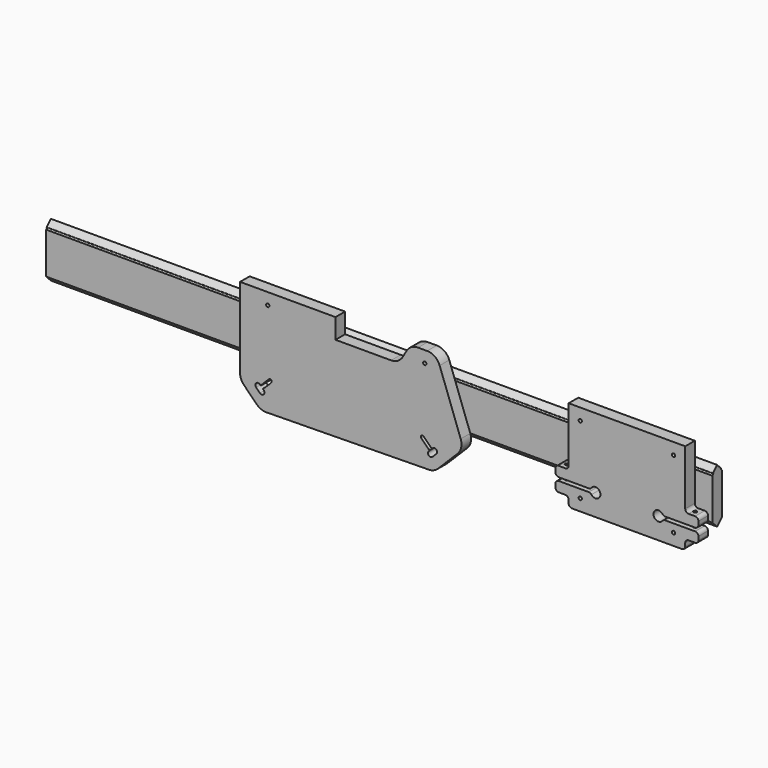
from build123d import *

# Parameters (mm, degrees)
F1_W      = 18
F1_H      = 80
F2_DEPTH  = 1000
F3_SIZE   = 8.99999
F5_DEPTH  = 1000
F6_R      = 2.5
F6_W      = 19.7983827577
F6_H      = 35
F7_DEPTH  = 18
F9_DEPTH  = 25
F10_R     = 5
F11_R     = 2.5
F12_DEPTH = 49.7830446156
F13_R     = 2.5
F14_DEPTH = 18
F15_R     = 20
F16_R     = 1


# Not quite as in the source:
# - a fillet or chamfer is up to 0.001 mm smaller than in the source, because OpenCascade refuses the exact size


with BuildPart() as f2:
    # F1 (on Right) → F2 (new body)
    with BuildSketch(Plane.YZ):
        with Locations((-9, 40)):
            Rectangle(F1_W, F1_H)
    extrude(amount=F2_DEPTH)

    # F3 (size 9 in the source; OpenCascade refuses exactly that, so slightly less here)
    f3_edges = [f2.edges().sort_by_distance(p)[0] for p in [
        (500, -18, 80),
        (500, 0, 80),
        (500, 0, 0),
        (500, -18, 0),
    ]]
    chamfer(f3_edges, length=F3_SIZE)


with BuildPart() as f5:
    # F4 (on face) → F5 (new body)
    with BuildSketch(Plane.YZ.offset(1000)):
        Polygon((-16.9195959493, 73.7774603256), (-16.0710678119, 72.9289321881), (-9, 80), (-1.9289321881, 72.9289321881), (-1.0804040507, 73.7774603256), (-9, 81.6970562748), align=None)
    extrude(amount=-F5_DEPTH)


with BuildPart() as f7:
    # F6 (on face) → F7 (new body)
    with BuildSketch(Plane.XZ.offset(18)):
        Polygon((973.7469878183, 108.6970562748), (798.7469878183, 108.6970562748), (798.7469878183, 21.0849883407), (798.7469878183, -13.9150116593), (798.7469878183, -28.6970562748), (973.7469878183, -28.6970562748), (973.7469878183, -13.9150116593), (973.7469878183, 21.0849883407), align=None)
        with Locations((816.2469878183, -11.1970562748)):
            Circle(F6_R, mode=Mode.SUBTRACT)
        with Locations((956.2469878183, -11.1970562748)):
            Circle(F6_R, mode=Mode.SUBTRACT)
        with Locations((816.2469878183, 91.1970562748)):
            Circle(F6_R, mode=Mode.SUBTRACT)
        with Locations((956.2469878183, 91.1970562748)):
            Circle(F6_R, mode=Mode.SUBTRACT)
        with Locations((788.8477964394, 3.5849883407)):
            Rectangle(F6_W, F6_H)
        with Locations((983.6461791972, 3.5849883407)):
            Rectangle(F6_W, F6_H)
    extrude(amount=F7_DEPTH)

    # F8 (on face) → F9 (cut)
    with BuildSketch(Plane.XZ.offset(36)):
        with BuildLine():
            Line((831.8775372487, 6.0849883407), (778.9486050606, 6.0849883407))
            Line((778.9486050606, 6.0849883407), (778.9486050606, 1.0849883407))
            Line((778.9486050606, 1.0849883407), (831.8775372487, 1.0849883407))
            ThreePointArc((831.8775372487, 1.0849883407), (831.4486050606, 3.5849883407), (831.8775372487, 6.0849883407))
        make_face()
        with BuildLine():
            ThreePointArc((846.4486050606, 3.5849883407), (840.216869901, 10.9769775381), (831.8775372487, 6.0849883407))
            Line((831.8775372487, 6.0849883407), (838.9486050606, 6.0849883407))
            Line((838.9486050606, 6.0849883407), (838.9486050606, 1.0849883407))
            Line((838.9486050606, 1.0849883407), (831.8775372487, 1.0849883407))
            ThreePointArc((831.8775372487, 1.0849883407), (840.216869901, -3.8070008567), (846.4486050606, 3.5849883407))
        make_face()
        with BuildLine():
            Line((838.9486050606, 6.0849883407), (831.8775372487, 6.0849883407))
            ThreePointArc((831.8775372487, 6.0849883407), (831.4486050606, 3.5849883407), (831.8775372487, 1.0849883407))
            Line((831.8775372487, 1.0849883407), (838.9486050606, 1.0849883407))
            Line((838.9486050606, 1.0849883407), (838.9486050606, 6.0849883407))
        make_face()
        with BuildLine():
            Line((940.6164383879, 6.0849883407), (933.5453705761, 6.0849883407))
            Line((933.5453705761, 6.0849883407), (933.5453705761, 1.0849883407))
            Line((933.5453705761, 1.0849883407), (940.6164383879, 1.0849883407))
            ThreePointArc((940.6164383879, 1.0849883407), (940.9373597735, 2.3167235003), (941.0453705761, 3.5849883407))
            ThreePointArc((941.0453705761, 3.5849883407), (940.9373597735, 4.8532531812), (940.6164383879, 6.0849883407))
        make_face()
        with BuildLine():
            Line((933.5453705761, 1.0849883407), (933.5453705761, 6.0849883407))
            Line((933.5453705761, 6.0849883407), (940.6164383879, 6.0849883407))
            ThreePointArc((940.6164383879, 6.0849883407), (926.0453705761, 3.5849883407), (940.6164383879, 1.0849883407))
            Line((940.6164383879, 1.0849883407), (933.5453705761, 1.0849883407))
        make_face()
        with BuildLine():
            Line((993.5453705761, 6.0849883407), (940.6164383879, 6.0849883407))
            ThreePointArc((940.6164383879, 6.0849883407), (940.9373597735, 4.8532531812), (941.0453705761, 3.5849883407))
            ThreePointArc((941.0453705761, 3.5849883407), (940.9373597735, 2.3167235003), (940.6164383879, 1.0849883407))
            Line((940.6164383879, 1.0849883407), (993.5453705761, 1.0849883407))
            Line((993.5453705761, 1.0849883407), (993.5453705761, 6.0849883407))
        make_face()
    extrude(amount=-F9_DEPTH, mode=Mode.SUBTRACT)

    # F10
    f10_edges = [f7.edges().sort_by_distance(p)[0] for p in [
        (778.948605, -27, 21.084988),
        (798.746988, -27, 21.084988),
        (778.948605, -27, 6.084988),
        (778.948605, -27, 1.084988),
        (831.877537, -27, 1.084988),
        (831.877537, -27, 6.084988),
        (940.616438, -27, 6.084988),
        (993.545371, -27, 6.084988),
        (993.545371, -27, 21.084988),
        (993.545371, -27, 1.084988),
        (973.746988, -27, 21.084988),
        (940.616438, -27, 1.084988),
        (798.746988, -27, -13.915012),
        (798.746988, -27, -28.697056),
        (973.746988, -27, -28.697056),
        (973.746988, -27, -13.915012),
        (993.545371, -27, -13.915012),
        (778.948605, -27, -13.915012),
    ]]
    fillet(f10_edges, radius=F10_R)

    # F11 (on face) → F12 (cut, through all)
    with BuildSketch(Plane.XY.offset(21.0849883407)):
        with Locations((788.8477964394, -27)):
            Circle(F11_R)
        with Locations((981.2469878183, -27)):
            Circle(F11_R)
    extrude(amount=-F12_DEPTH, mode=Mode.SUBTRACT)


with BuildPart() as f14:
    # F13 (on face) → F14 (new body)
    with BuildSketch(Plane.XZ.offset(18)):
        Polygon((448.7895516693, 108.6970562748), (305.5662543474, 108.6970562748), (305.5662543474, -19.9349505144), (336.6135691666, -50.9822653337), (596.9457328866, -47.2548845621), (641.0791762714, -3.1214411773), (600.3805715585, 108.6970562748), (561.1554156828, 108.6970562748), (543.8349076071, 78.6970562748), (448.7895516693, 78.6970562748), align=None)
        with BuildLine():
            Line((338.3023187565, -20.144102989), (341.018998398, -22.8607826305))
            ThreePointArc((341.018998398, -22.8607826305), (341.018998398, -28.51763688), (335.3621441485, -28.51763688))
            Line((335.3621441485, -28.51763688), (329.705289899, -22.8607826305))
            ThreePointArc((329.705289899, -22.8607826305), (329.705289899, -17.203928381), (335.3621441485, -17.203928381))
            Line((335.3621441485, -17.203928381), (338.0788237901, -19.9206080226))
            ThreePointArc((338.0788237901, -19.9206080226), (337.456053005, -18.1890671452), (338.1870357394, -16.5003571337))
            Line((338.1870357394, -16.5003571337), (348.7936374572, -5.8937554159))
            ThreePointArc((348.7936374572, -5.8937554159), (351.518112991, -5.3518235376), (353.0614044101, -7.6615223689))
            ThreePointArc((353.0614044101, -7.6615223689), (352.8711032414, -8.6182309498), (352.3291713631, -9.4292893219))
            Line((352.3291713631, -9.4292893219), (341.7225696453, -20.0358910397))
            ThreePointArc((341.7225696453, -20.0358910397), (340.0338596338, -20.7668737741), (338.3023187565, -20.144102989))
        make_face(mode=Mode.SUBTRACT)
        with BuildLine():
            ThreePointArc((591.6448855423, -16.5003571337), (592.1868174206, -17.3114155058), (592.3771185893, -18.2681240867))
            ThreePointArc((592.3771185893, -18.2681240867), (592.215916064, -19.1513151035), (591.7530974916, -19.9206080226))
            Line((591.7530974916, -19.9206080226), (594.4697771331, -17.203928381))
            ThreePointArc((594.4697771331, -17.203928381), (600.1266313826, -17.203928381), (600.1266313826, -22.8607826305))
            Line((600.1266313826, -22.8607826305), (594.4697771331, -28.51763688))
            ThreePointArc((594.4697771331, -28.51763688), (588.8129228836, -28.51763688), (588.8129228836, -22.8607826305))
            Line((588.8129228836, -22.8607826305), (591.5296025252, -20.144102989))
            ThreePointArc((591.5296025252, -20.144102989), (589.7980616478, -20.7668737741), (588.1093516363, -20.0358910397))
            Line((588.1093516363, -20.0358910397), (577.5027499185, -9.4292893219))
            ThreePointArc((577.5027499185, -9.4292893219), (577.5027499185, -5.8937554159), (581.0382838245, -5.8937554159))
            Line((581.0382838245, -5.8937554159), (591.6448855423, -16.5003571337))
        make_face(mode=Mode.SUBTRACT)
        with Locations((347.0258705042, 91.1970562748)):
            Circle(F13_R, mode=Mode.SUBTRACT)
        with Locations((582.8060507774, 91.1970562748)):
            Circle(F13_R, mode=Mode.SUBTRACT)
    extrude(amount=F14_DEPTH)

    # F15
    f15_edges = [f14.edges().sort_by_distance(p)[0] for p in [
        (561.155416, -27, 108.697056),
        (600.380572, -27, 108.697056),
        (543.834908, -27, 78.697056),
        (596.945733, -27, -47.254885),
        (336.613569, -27, -50.982265),
        (305.566254, -27, -19.934951),
        (641.079176, -27, -3.121441),
    ]]
    fillet(f15_edges, radius=F15_R)

    # F16
    f16_edges = [f14.edges().sort_by_distance(p)[0] for p in [
        (338.302319, -27, -20.144103),
        (338.078824, -27, -19.920608),
        (591.753097, -27, -19.920608),
        (591.529603, -27, -20.144103),
    ]]
    fillet(f16_edges, radius=F16_R)


solid = Compound([f2.part, f5.part, f7.part, f14.part])
